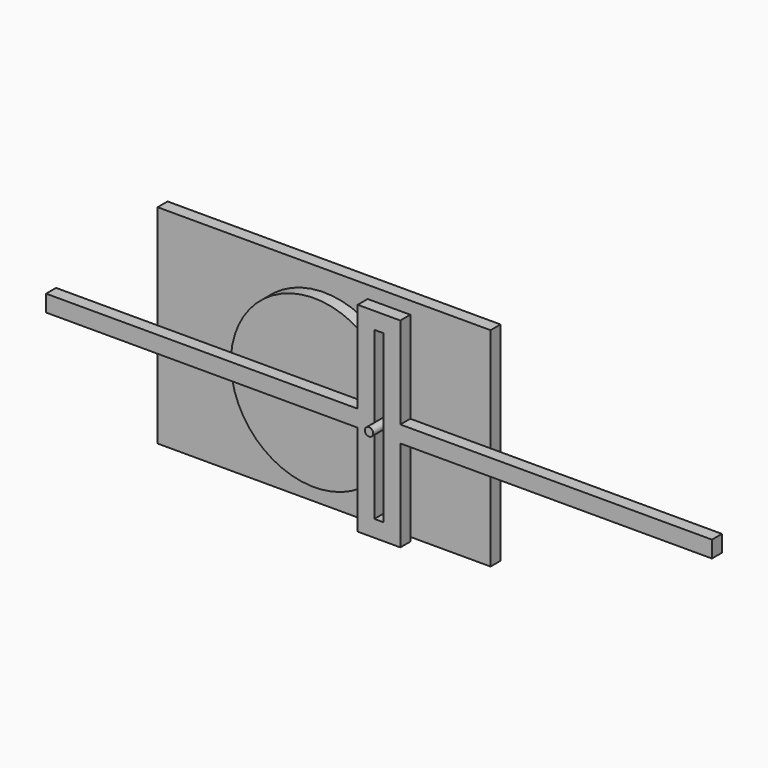
from build123d import *

# Parameters (mm, degrees)
F1_R     = 63.5
F1_R_2   = 3.3782
F2_DEPTH = 9.525
F3_R     = 3.175
F4_DEPTH = 19.05
F3_W     = 12.6873
F3_H     = 12.7
F3_W_2   = 237.7313
F5_DEPTH = 9.525
F6_W     = 254
F6_H     = 158.75
F6_R     = 63.5
F6_R_2   = 3.3782
F7_DEPTH = 9.525


with BuildPart() as f2:
    # F1 (on Front) → F2 (new body)
    with BuildSketch(Plane.XZ):
        Circle(F1_R)
        Circle(F1_R_2, mode=Mode.SUBTRACT)
    extrude(amount=F2_DEPTH)

    # F3 (on face) → F4 (join)
    with BuildSketch(Plane.XZ.offset(9.525)):
        with Locations((57.15, 0)):
            Circle(F3_R)
    extrude(amount=F4_DEPTH)


with BuildPart() as f5:
    # F3 (on face) → F5 (new body)
    with BuildSketch(Plane.XZ.offset(9.525)):
        Polygon((53.5686, 6.35), (53.5686, 63.5), (60.7314, 63.5), (60.7314, 6.35), (73.4187, 6.35), (73.4187, 76.2), (40.8813, 76.2), (40.8813, 6.35), align=None)
        with Locations((47.22495, 0)):
            Rectangle(F3_W, F3_H)
        with Locations((67.07505, 0)):
            Rectangle(F3_W, F3_H)
        Polygon((53.5686, -63.5), (53.5686, -6.35), (40.8813, -6.35), (40.8813, -76.2), (73.4187, -76.2), (73.4187, -6.35), (60.7314, -6.35), (60.7314, -63.5), align=None)
        with Locations((-77.98435, 0)):
            Rectangle(F3_W_2, F3_H)
        with Locations((192.28435, 0)):
            Rectangle(F3_W_2, F3_H)
    extrude(amount=F5_DEPTH)


with BuildPart() as f7:
    # F6 (on face) → F7 (new body)
    with BuildSketch(Plane(origin=(0, 0, 0), x_dir=(-1, 0, 0), z_dir=(0, 1, 0))):
        Rectangle(F6_W, F6_H)
        Circle(F6_R, mode=Mode.SUBTRACT)
        Circle(F6_R)
        Circle(F6_R_2, mode=Mode.SUBTRACT)
    extrude(amount=F7_DEPTH)


solid = Compound([f2.part, f5.part, f7.part])
